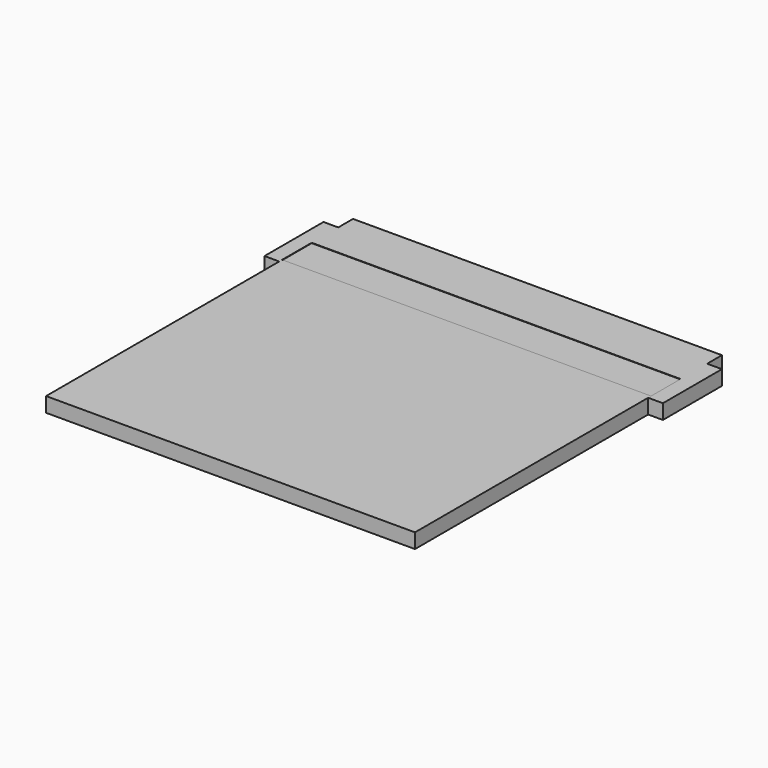
from build123d import *

# Parameters (mm, degrees)
F1_DEPTH = 4
F2_W     = 100
F2_H     = 10
F3_DEPTH = 0.1


# Not quite as in the source:
# - a feature names something its author has since deleted; it is built from what else it names


with BuildPart() as f1:
    # F0 (on Top) → F1 (new body)
    with BuildSketch(Plane.XY):
        Polygon((-50, -49.5), (50, -49.5), (50, 29.5), (54, 29.5), (54, 49.5), (50, 49.5), (50, 54.5), (-50, 54.5), (-50, 49.5), (-54, 49.5), (-54, 29.5), (-50, 29.5), align=None)
    extrude(amount=F1_DEPTH)

    # F2 (on face) → F3 (cut)
    with BuildSketch(Plane.XY.offset(4)):
        with Locations((0, 35.5)):
            Rectangle(F2_W, F2_H)
    extrude(amount=-F3_DEPTH, mode=Mode.SUBTRACT)


solid = f1.part
